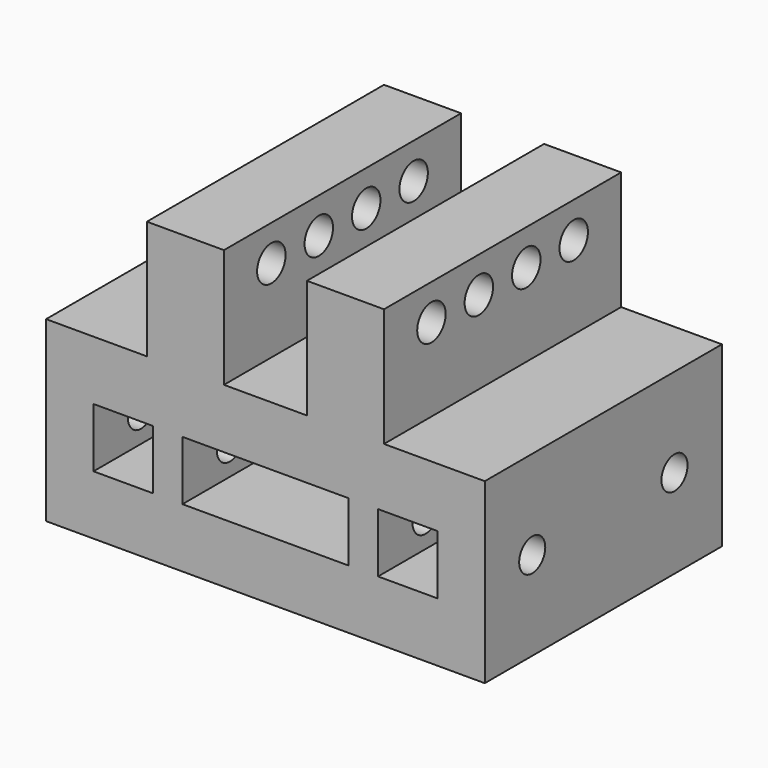
from build123d import *

# Parameters (mm, degrees)
F0_W     = 5
F0_H     = 5
F0_W_2   = 14
F0_W_3   = 6.5
F0_H_2   = 10
F1_DEPTH = 25
F2_R     = 1.5
F3_DEPTH = 37


with BuildPart() as f1:
    # F0 (on Front) → F1 (new body)
    with BuildSketch(Plane.XZ):
        Polygon((-18.5, -7.5), (18.5, -7.5), (18.5, 7.5), (10, 7.5), (3.5, 7.5), (-3.5, 7.5), (-10, 7.5), (-18.5, 7.5), align=None)
        with Locations((-12, 0)):
            Rectangle(F0_W, F0_H, mode=Mode.SUBTRACT)
        Rectangle(F0_W_2, F0_H, mode=Mode.SUBTRACT)
        with Locations((12, 0)):
            Rectangle(F0_W, F0_H, mode=Mode.SUBTRACT)
        with Locations((6.75, 12.5)):
            Rectangle(F0_W_3, F0_H_2)
        with Locations((-6.75, 12.5)):
            Rectangle(F0_W_3, F0_H_2)
    extrude(amount=F1_DEPTH)

    # F2 (on face) → F3 (cut, through all)
    with BuildSketch(Plane(origin=(-18.5, 0, 0), x_dir=(0, -1, 0), z_dir=(-1, 0, 0))):
        with Locations((5, 14.5)):
            Circle(F2_R)
        with Locations((10, 14.5)):
            Circle(F2_R)
        with Locations((15, 14.5)):
            Circle(F2_R)
        with Locations((20, 14.5)):
            Circle(F2_R)
        with BuildLine():
            Line((18.625, 0), (21.375, 0))
            ThreePointArc((21.375, 0), (20, 1.375), (18.625, 0))
        make_face()
        with BuildLine():
            Line((3.625, 0), (6.375, 0))
            ThreePointArc((6.375, 0), (5, 1.375), (3.625, 0))
        make_face()
        with BuildLine():
            ThreePointArc((3.625, 0), (5, -1.375), (6.375, 0))
            Line((6.375, 0), (3.625, 0))
        make_face()
        with BuildLine():
            ThreePointArc((18.625, 0), (20, -1.375), (21.375, 0))
            Line((21.375, 0), (18.625, 0))
        make_face()
    extrude(amount=-F3_DEPTH, mode=Mode.SUBTRACT)


solid = f1.part
